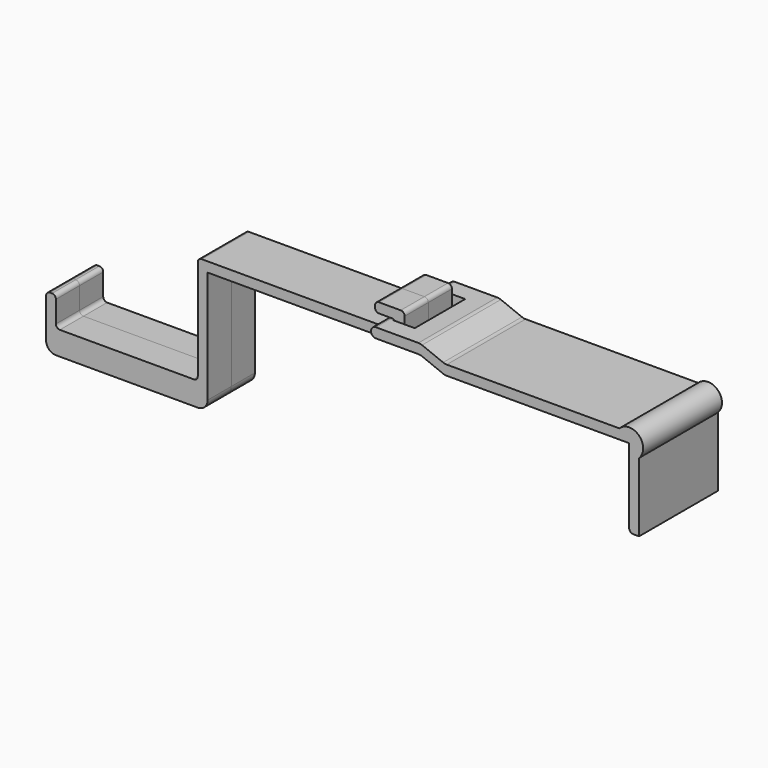
from build123d import *

# Parameters (mm, degrees)
F1_DEPTH      = 15
F1_DEPTH_BACK = 15
F0_W          = 5.9289547801
F0_H          = 5
F2_DEPTH      = 25
F2_DEPTH_BACK = 25
F3_DEPTH      = 16
F3_DEPTH_BACK = 16
F4_DEPTH      = 10
F4_DEPTH_BACK = 10


with BuildPart() as f1:
    # F0 (on Front) → F1 (new body, two sides)
    with BuildSketch(Plane.XZ) as f1_sk:
        with BuildLine():
            Line((-18.1352669001, 5), (-111.5642216802, 5))
            Line((-111.5642216802, 5), (-114.5642216802, 5))
            ThreePointArc((-114.5642216802, 5), (-115.9784352425, 4.4142135624), (-116.5642216802, 3))
            Line((-116.5642216802, 3), (-116.5642216802, -48))
            ThreePointArc((-116.5642216802, -48), (-117.1500081178, -49.4142135624), (-118.5642216802, -50))
            Line((-118.5642216802, -50), (-186.5642216802, -50))
            ThreePointArc((-186.5642216802, -50), (-187.9784352425, -49.4142135624), (-188.5642216802, -48))
            Line((-188.5642216802, -48), (-188.5642216802, -37))
            ThreePointArc((-188.5642216802, -37), (-189.1500081178, -35.5857864376), (-190.5642216802, -35))
            Line((-190.5642216802, -35), (-191.5642216802, -35))
            ThreePointArc((-191.5642216802, -35), (-192.9784352425, -35.5857864376), (-193.5642216802, -37))
            Line((-193.5642216802, -37), (-193.5642216802, -50))
            Line((-193.5642216802, -50), (-193.5642216802, -57))
            ThreePointArc((-193.5642216802, -57), (-192.0997555861, -60.5355339059), (-188.5642216802, -62))
            Line((-188.5642216802, -62), (-116.5642216802, -62))
            ThreePointArc((-116.5642216802, -62), (-113.0286877742, -60.5355339059), (-111.5642216802, -57))
            Line((-111.5642216802, -57), (-111.5642216802, -50))
            Line((-111.5642216802, -50), (-111.5642216802, 0))
            Line((-111.5642216802, 0), (-13.5642216802, 0))
            ThreePointArc((-13.5642216802, 0), (-12.1500081178, 0.5857864376), (-11.5642216802, 2))
            Line((-11.5642216802, 2), (-11.5642216802, 5))
            Line((-11.5642216802, 5), (-15.6352669001, 5))
            Line((-15.6352669001, 5), (-18.1352669001, 5))
        make_face()
        with BuildLine():
            Line((-24.5642216802, 10), (-18.1352669001, 10))
            Line((-18.1352669001, 10), (-15.6352669001, 10))
            Line((-15.6352669001, 10), (-11.5642216802, 10))
            Line((-11.5642216802, 10), (-11.5642216802, 13))
            ThreePointArc((-11.5642216802, 13), (-12.1500081178, 14.4142135624), (-13.5642216802, 15))
            Line((-13.5642216802, 15), (-24.5642216802, 15))
            ThreePointArc((-24.5642216802, 15), (-25.9784352425, 14.4142135624), (-26.5642216802, 13))
            Line((-26.5642216802, 13), (-26.5642216802, 12))
            ThreePointArc((-26.5642216802, 12), (-25.9784352425, 10.5857864376), (-24.5642216802, 10))
        make_face()
        with BuildLine():
            Line((-15.6352669001, 10), (-18.1352669001, 10))
            ThreePointArc((-18.1352669001, 10), (-16.3674999471, 9.267766953), (-15.6352669001, 7.5))
            Line((-15.6352669001, 7.5), (-15.6352669001, 10))
        make_face()
        Polygon((-15.6352669001, 7.5), (-15.6352669001, 5), (-11.5642216802, 5), (-11.5642216802, 10), (-15.6352669001, 10), align=None)
        with BuildLine():
            ThreePointArc((-15.6352669001, 7.5), (-16.3674999471, 5.732233047), (-18.1352669001, 5))
            Line((-18.1352669001, 5), (-15.6352669001, 5))
            Line((-15.6352669001, 5), (-15.6352669001, 7.5))
        make_face()
    extrude(amount=F1_DEPTH)
    extrude(f1_sk.sketch, amount=-F1_DEPTH_BACK)


with BuildPart() as f2:
    # F0 (on Front) → F2 (new body, two sides)
    with BuildSketch(Plane.XZ) as f2_sk:
        with BuildLine():
            ThreePointArc((-18.1352669001, 10), (-20.6352669001, 7.5), (-18.1352669001, 5))
            Line((-18.1352669001, 5), (-18.1352669001, 10))
        make_face()
        with BuildLine():
            Line((-18.1352669001, 10), (-18.1352669001, 5))
            ThreePointArc((-18.1352669001, 5), (-16.3674999471, 5.732233047), (-15.6352669001, 7.5))
            ThreePointArc((-15.6352669001, 7.5), (-16.3674999471, 9.267766953), (-18.1352669001, 10))
        make_face()
        with BuildLine():
            Line((-15.6352669001, 10), (-18.1352669001, 10))
            ThreePointArc((-18.1352669001, 10), (-16.3674999471, 9.267766953), (-15.6352669001, 7.5))
            Line((-15.6352669001, 7.5), (-15.6352669001, 10))
        make_face()
        with BuildLine():
            ThreePointArc((-15.6352669001, 7.5), (-16.3674999471, 5.732233047), (-18.1352669001, 5))
            Line((-18.1352669001, 5), (-15.6352669001, 5))
            Line((-15.6352669001, 5), (-15.6352669001, 7.5))
        make_face()
        Polygon((-15.6352669001, 7.5), (-15.6352669001, 5), (-11.5642216802, 5), (-11.5642216802, 10), (-15.6352669001, 10), align=None)
        with Locations((-8.5997442901, 7.5)):
            Rectangle(F0_W, F0_H)
        with BuildLine():
            Line((-5.6352669001, 10), (-5.6352669001, 5))
            Line((-5.6352669001, 5), (3.4018210821, 5))
            ThreePointArc((3.4018210821, 5), (4.3473586879, 4.9097819337), (5.2587744639, 4.6423834544))
            Line((5.2587744639, 4.6423834544), (15.970691736, 0.3576165456))
            ThreePointArc((15.970691736, 0.3576165456), (16.882107512, 0.0902180663), (17.8276451178, 0))
            Line((17.8276451178, 0), (110.4357783198, 0))
            Line((110.4357783198, 0), (110.4357783198, -38))
            ThreePointArc((110.4357783198, -38), (111.0215647575, -39.4142135624), (112.4357783198, -40))
            Line((112.4357783198, -40), (115.4357783198, -40))
            Line((115.4357783198, -40), (115.4357783198, -5))
            ThreePointArc((115.4357783198, -5), (115.4357783198, 5), (105.4357783198, 5))
            Line((105.4357783198, 5), (17.8276451178, 5))
            ThreePointArc((17.8276451178, 5), (16.882107512, 5.0902180663), (15.970691736, 5.3576165456))
            Line((15.970691736, 5.3576165456), (5.2587744639, 9.6423834544))
            ThreePointArc((5.2587744639, 9.6423834544), (4.8179202782, 9.7952750773), (4.3647330999, 9.9064040239))
            ThreePointArc((4.3647330999, 9.9064040239), (3.8855461489, 9.976545997), (3.4018210821, 10))
            Line((3.4018210821, 10), (-5.6352669001, 10))
        make_face()
    extrude(amount=F2_DEPTH)
    extrude(f2_sk.sketch, amount=-F2_DEPTH_BACK)

    # F0 (on Front) → F3 (cut, two sides)
    with BuildSketch(Plane.XZ) as f3_sk:
        with BuildLine():
            Line((-15.6352669001, 10), (-18.1352669001, 10))
            ThreePointArc((-18.1352669001, 10), (-16.3674999471, 9.267766953), (-15.6352669001, 7.5))
            Line((-15.6352669001, 7.5), (-15.6352669001, 10))
        make_face()
        with BuildLine():
            ThreePointArc((-15.6352669001, 7.5), (-16.3674999471, 5.732233047), (-18.1352669001, 5))
            Line((-18.1352669001, 5), (-15.6352669001, 5))
            Line((-15.6352669001, 5), (-15.6352669001, 7.5))
        make_face()
        Polygon((-15.6352669001, 7.5), (-15.6352669001, 5), (-11.5642216802, 5), (-11.5642216802, 10), (-15.6352669001, 10), align=None)
        with Locations((-8.5997442901, 7.5)):
            Rectangle(F0_W, F0_H)
    extrude(amount=-F3_DEPTH, mode=Mode.SUBTRACT)
    extrude(f3_sk.sketch, amount=F3_DEPTH_BACK, mode=Mode.SUBTRACT)

    # F0 (on Front) → F4 (join, two sides)
    with BuildSketch(Plane.XZ) as f4_sk:
        with BuildLine():
            Line((3.4018210821, 5), (-5.6352669001, 5))
            add(Edge.make_bspline(
                [(-5.6352669001, 5), (4.3647330999, 5), (0, 0), (17.8276451178, 0)],
                knots=[0, 0, 0, 0, 23.9897528198, 23.9897528198, 23.9897528198, 23.9897528198], degree=3))
            ThreePointArc((17.8276451178, 0), (16.882107512, 0.0902180663), (15.970691736, 0.3576165456))
            Line((15.970691736, 0.3576165456), (5.2587744639, 4.6423834544))
            ThreePointArc((5.2587744639, 4.6423834544), (4.3473586879, 4.9097819337), (3.4018210821, 5))
        make_face()
    extrude(amount=F4_DEPTH)
    extrude(f4_sk.sketch, amount=-F4_DEPTH_BACK)


solid = Compound([f1.part, f2.part])
